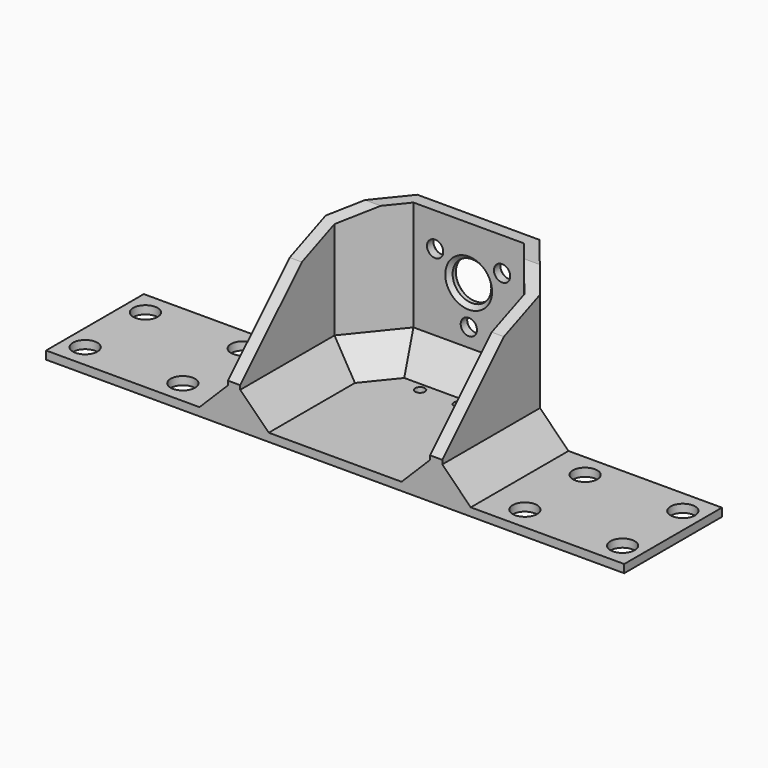
from build123d import *

# Parameters (mm, degrees)
F0_R         = 3
F1_DEPTH     = 2
F3_DEPTH     = 21
F4_R         = 2
F5_DEPTH     = 3
F6_DEPTH     = 44.001
F7_SIZE      = 7
F8_DEPTH     = 13
F9_SIZE      = 26
F10_T1_DEPTH = 54.8534078581
F10_T3_DEPTH = 54.8534078581
F11_SIZE     = 8
F12_SIZE     = 1
F13_SIZE     = 1
F14_R        = 1.2
F15_DEPTH    = 2


# Not quite as in the source:
# - a fillet or chamfer that OpenCascade refuses, or shapes differently, is made with other operations: its cross-section is extruded or revolved along the edge and cut away or added


with BuildPart() as f1:
    # F0 (on Top) → F1 (new body)
    with BuildSketch(Plane.XY):
        Polygon((-71, -15), (71, -15), (71, 15), (26.313708499, 15), (15, 29), (-15, 29), (-26.313708499, 15), (-71, 15), align=None)
        with Locations((-66, -9.25)):
            Circle(F0_R, mode=Mode.SUBTRACT)
        with Locations((-42, -9.25)):
            Circle(F0_R, mode=Mode.SUBTRACT)
        with Locations((42, -9.25)):
            Circle(F0_R, mode=Mode.SUBTRACT)
        with Locations((66, -9.25)):
            Circle(F0_R, mode=Mode.SUBTRACT)
        with Locations((-66, 9.25)):
            Circle(F0_R, mode=Mode.SUBTRACT)
        with Locations((-42, 9.25)):
            Circle(F0_R, mode=Mode.SUBTRACT)
        with Locations((42, 9.25)):
            Circle(F0_R, mode=Mode.SUBTRACT)
        with Locations((66, 9.25)):
            Circle(F0_R, mode=Mode.SUBTRACT)
    extrude(amount=F1_DEPTH)

    # F2 (on face) → F3 (join)
    with BuildSketch(Plane.XY.offset(2)):
        Polygon((-15, 29), (-26.313708499, 15), (-26.313708499, -15), (-23.313708499, -15), (-23.313708499, 13.9393398282), (-13.5672232498, 26), (13.5672232498, 26), (23.313708499, 13.9393398282), (23.313708499, -15), (26.313708499, -15), (26.313708499, 15), (15, 29), align=None)
    extrude(amount=F3_DEPTH)

    # F4 (on face) → F5 (join)
    with BuildSketch(Plane(origin=(0, 29, 0), x_dir=(-1, 0, 0), z_dir=(0, 1, 0))):
        with BuildLine():
            ThreePointArc((-4.75, 23), (0, 27.75), (4.75, 23))
            Line((4.75, 23), (15, 23))
            Line((15, 23), (15, 36))
            Line((15, 36), (0, 36))
            Line((0, 36), (-15, 36))
            Line((-15, 36), (-15, 23))
            Line((-15, 23), (-4.75, 23))
        make_face()
        with Locations((-8.2078662679, 27.7834016482)):
            Circle(F4_R, mode=Mode.SUBTRACT)
        with Locations((8.2464804778, 27.7165198748)):
            Circle(F4_R, mode=Mode.SUBTRACT)
    extrude(amount=-F5_DEPTH)

    # F4 (on face) → F6 (cut, through all)
    with BuildSketch(Plane(origin=(0, 29, 0), x_dir=(-1, 0, 0), z_dir=(0, 1, 0))):
        with Locations((-8.2078662679, 27.7834016482)):
            Circle(F4_R)
        with BuildLine():
            ThreePointArc((-4.75, 23), (0, 18.25), (4.75, 23))
            Line((4.75, 23), (-4.75, 23))
        make_face()
        with Locations((-0.0386142099, 13.500078477)):
            Circle(F4_R)
    extrude(amount=-F6_DEPTH, mode=Mode.SUBTRACT)

    # F7
    f7_edges = [f1.edges().sort_by_distance(p)[0] for p in [
        (-26.313708, 0, 2),
        (23.313708, -0.53033, 2),
        (18.440466, 19.96967, 2),
        (-18.440466, 19.96967, 2),
        (-23.313708, -0.53033, 2),
        (26.313708, 0, 2),
        (0, 26, 2),
        (0, 29, 0),
    ]]
    chamfer(f7_edges, length=F7_SIZE)

    # F8 (add): faces of the model
    f8_faces = [f1.faces().sort_by_distance(p)[0] for p in [
        (-15.4580909174, 27.5, 23),
        (25.8556175816, 0, 23),
    ]]
    extrude(f8_faces, amount=F8_DEPTH)

    # F9
    f9_edges = [f1.edges().sort_by_distance(p)[0] for p in [
        (-24.813708, -15, 36),
        (24.813708, -15, 36),
    ]]
    chamfer(f9_edges, length=F9_SIZE)

    # F10: chamfer of 10 on 2 edges, made by hand

    # F10_s2 → F10_t1 (cut)
    with BuildSketch(Plane.YZ.offset(-52.2404124281)):
        Polygon((3.9289321881, 28.9289321881), (21, 36), (11, 36), align=None)
    extrude(amount=F10_T1_DEPTH, mode=Mode.SUBTRACT)

    # F10_s4 → F10_t3 (cut)
    with BuildSketch(Plane.YZ.offset(-2.6129954301)):
        Polygon((3.9289321881, 28.9289321881), (21, 36), (11, 36), align=None)
    extrude(amount=F10_T3_DEPTH, mode=Mode.SUBTRACT)

    # F11
    f11_edges = [f1.edges().sort_by_distance(p)[0] for p in [
        (23.485281, 18.5, 0),
        (-23.485281, 18.5, 0),
    ]]
    chamfer(f11_edges, length=F11_SIZE)

    # F12
    f12_edges = [f1.edges().sort_by_distance(p)[0] for p in [
        (2.038614, 29, 13.500078),
        (10.207866, 29, 27.783402),
        (-6.24648, 29, 27.71652),
    ]]
    chamfer(f12_edges, length=F12_SIZE)

    # F13
    f13_edges = [f1.edges().sort_by_distance(p)[0] for p in [
        (-4.75, 26, 23),
        (-4.75, 29, 23),
    ]]
    chamfer(f13_edges, length=F13_SIZE)

    # F14 (on face) → F15 (cut, through all)
    with BuildSketch(Plane(origin=(0, 0, 0), x_dir=(1, 0, 0), z_dir=(0, 0, -1))):
        with Locations((-4.75, -17)):
            Circle(F14_R)
        with BuildLine():
            ThreePointArc((5.95, -17), (4.75, -15.8), (3.55, -17))
            ThreePointArc((3.55, -17), (4.75, -18.2), (5.95, -17))
        make_face()
    extrude(amount=-F15_DEPTH, mode=Mode.SUBTRACT)


solid = f1.part
